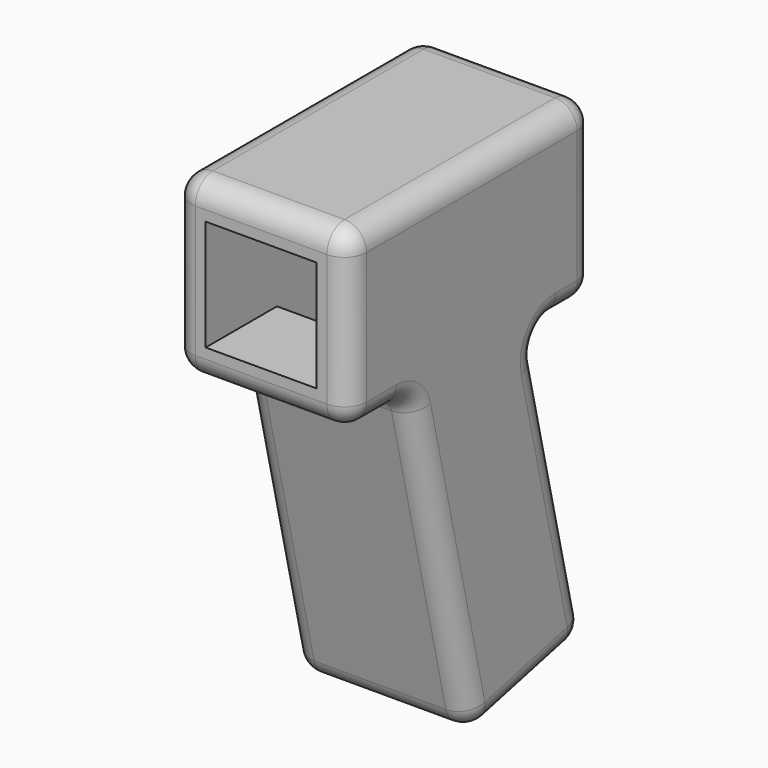
from build123d import *

# Parameters (mm, degrees)
F1_DEPTH      = 8
F2_W          = 10.1
F2_H          = 10.1
F3_DEPTH      = 28
F4_W          = 10.1
F4_H          = 10.1
F5_DEPTH      = 33.3776100313
F6_T1_DEPTH   = 16
F6_T3_DEPTH   = 12
F6_T5_DEPTH   = 24
F6_T7_DEPTH   = 19
F6_T9_DEPTH   = 23.6326677566
F6_T11_DEPTH  = 26
F6_S15_W      = 2
F6_S15_H      = 2
F6_T16_DEPTH  = 2
F6_S21_W      = 2
F6_S21_H      = 2
F6_T22_DEPTH  = 2
F6_S27_W      = 2
F6_S27_H      = 2
F6_T28_DEPTH  = 2
F6_S33_W      = 2
F6_S33_H      = 2
F6_T34_DEPTH  = 2
F6_T37_DEPTH  = 23.0526598256
F6_T39_DEPTH  = 2.4787085237
F6_T41_DEPTH  = 3.4135114731
F6_T43_DEPTH  = 27.1734272819
F6_S47_W      = 2
F6_S47_H      = 2
F6_T48_DEPTH  = 2
F6_S53_W      = 2
F6_S53_H      = 2
F6_T54_DEPTH  = 2
F6_S59_W      = 2
F6_S59_H      = 2
F6_T60_DEPTH  = 2
F6_T66_DEPTH  = 2
F6_T72_DEPTH  = 2
F6_S77_W      = 2
F6_S77_H      = 2
F6_T78_DEPTH  = 2
F6_S83_W      = 2
F6_S83_H      = 2
F6_T84_DEPTH  = 2
F6_S89_W      = 2
F6_S89_H      = 2
F6_T90_DEPTH  = 2
F6_T94_ANGLE  = 76.8460155346
F6_T96_ANGLE  = 103.1539844654
F6_T98_ANGLE  = 76.8460155346
F6_T100_ANGLE = 103.1539844654


# Not quite as in the source:
# - a fillet or chamfer that OpenCascade refuses, or shapes differently, is made with other operations: its cross-section is extruded or revolved along the edge and cut away or added


with BuildPart() as f1:
    # F0 (on Right) → F1 (new body, symmetric)
    with BuildSketch(Plane.YZ):
        Polygon((7, -8), (14, -8), (14, 8), (-14, 8), (-14, -8), (-7, -8), (0, -37.9528366029), (13.2749735829, -34.8504654882), align=None)
    extrude(amount=F1_DEPTH, both=True)

    # F2 (on face) → F3 (cut, through all)
    with BuildSketch(Plane(origin=(0, 14, 0), x_dir=(-1, 0, 0), z_dir=(0, 1, 0))):
        Rectangle(F2_W, F2_H)
    extrude(amount=-F3_DEPTH, mode=Mode.SUBTRACT)

    # F4 (on face) → F5 (cut, through all)
    with BuildSketch(Plane(origin=(0, 8.4102702856, -35.9873502358), x_dir=(1, 0, 0), z_dir=(0, 0.2275688933, -0.9737619826))):
        with Locations((0, 1.8205511468)):
            Rectangle(F4_W, F4_H)
    extrude(amount=-F5_DEPTH, mode=Mode.SUBTRACT)

    # F6: fillet of radius 2 on 24 edges, made by hand

    # F6_s2 → F6_t1 (join)
    with BuildSketch(Plane.YZ.offset(-8)):
        with BuildLine():
            ThreePointArc((-8.5864885269, -8), (-7.3435636646, -8.4331120695), (-6.6389645616, -9.5448622133))
            Line((-6.6389645616, -9.5448622133), (-7, -8))
            Line((-7, -8), (-8.5864885269, -8))
        make_face()
        with BuildLine():
            ThreePointArc((7.5737675111, -10.4551377867), (7.9544035458, -8.7570751377), (9.5212914763, -8))
            Line((9.5212914763, -8), (7, -8))
            Line((7, -8), (7.5737675111, -10.4551377867))
        make_face()
    extrude(amount=F6_T1_DEPTH)

    # F6_s4 → F6_t3 (cut)
    with BuildSketch(Plane.YZ.offset(-6)):
        with BuildLine():
            ThreePointArc((14, 6), (13.4142135624, 7.4142135624), (12, 8))
            Line((12, 8), (14, 8))
            Line((14, 8), (14, 6))
        make_face()
        with BuildLine():
            ThreePointArc((-12, 8), (-13.4142135624, 7.4142135624), (-14, 6))
            Line((-14, 6), (-14, 8))
            Line((-14, 8), (-12, 8))
        make_face()
    extrude(amount=F6_T3_DEPTH, mode=Mode.SUBTRACT)

    # F6_s6 → F6_t5 (cut)
    with BuildSketch(Plane.XZ.offset(-12)):
        with BuildLine():
            ThreePointArc((-8, 6), (-7.4142135624, 7.4142135624), (-6, 8))
            Line((-6, 8), (-8, 8))
            Line((-8, 8), (-8, 6))
        make_face()
        with BuildLine():
            ThreePointArc((8, 6), (7.4142135624, 7.4142135624), (6, 8))
            Line((6, 8), (8, 8))
            Line((8, 8), (8, 6))
        make_face()
    extrude(amount=F6_T5_DEPTH, mode=Mode.SUBTRACT)

    # F6_s8 → F6_t7 (cut)
    with BuildSketch(Plane.XY.offset(-13)):
        with BuildLine():
            ThreePointArc((-8, 12), (-7.4142135624, 13.4142135624), (-6, 14))
            Line((-6, 14), (-8, 14))
            Line((-8, 14), (-8, 12))
        make_face()
        with BuildLine():
            ThreePointArc((-8, -12), (-7.4142135624, -13.4142135624), (-6, -14))
            Line((-6, -14), (-8, -14))
            Line((-8, -14), (-8, -12))
        make_face()
        with BuildLine():
            ThreePointArc((8, 12), (7.4142135624, 13.4142135624), (6, 14))
            Line((6, 14), (8, 14))
            Line((8, 14), (8, 12))
        make_face()
        with BuildLine():
            ThreePointArc((8, -12), (7.4142135624, -13.4142135624), (6, -14))
            Line((6, -14), (8, -14))
            Line((8, -14), (8, -12))
        make_face()
    extrude(amount=F6_T7_DEPTH, mode=Mode.SUBTRACT)

    # F6_s10 → F6_t9 (cut)
    with BuildSketch(Plane(origin=(0, -13.2790801987, -3.1033308338), x_dir=(1, 0, 0), z_dir=(0, 0.9737619826, 0.2275688933))):
        with BuildLine():
            ThreePointArc((-6, 36.9570294162), (-7.4142135624, 36.3712429786), (-8, 34.9570294162))
            Line((-8, 34.9570294162), (-8, 36.9570294162))
            Line((-8, 36.9570294162), (-6, 36.9570294162))
        make_face()
        with BuildLine():
            ThreePointArc((6, 36.9570294162), (7.4142135624, 36.3712429786), (8, 34.9570294162))
            Line((8, 34.9570294162), (8, 36.9570294162))
            Line((8, 36.9570294162), (6, 36.9570294162))
        make_face()
    extrude(amount=F6_T9_DEPTH, mode=Mode.SUBTRACT)

    # F6_s12 → F6_t11 (cut)
    with BuildSketch(Plane.YZ.offset(-13)):
        with BuildLine():
            ThreePointArc((1.9475239652, -37.4976988162), (0.4371097915, -37.2491132687), (-0.4551377867, -36.0053126377))
            Line((-0.4551377867, -36.0053126377), (0, -37.9528366029))
            Line((0, -37.9528366029), (1.9475239652, -37.4976988162))
        make_face()
        with BuildLine():
            ThreePointArc((12.8198357962, -32.902941523), (12.5712502487, -34.4133556967), (11.3274496177, -35.3056032749))
            Line((11.3274496177, -35.3056032749), (13.2749735829, -34.8504654882))
            Line((13.2749735829, -34.8504654882), (12.8198357962, -32.902941523))
        make_face()
        with BuildLine():
            ThreePointArc((12, -8), (13.4142135624, -7.4142135624), (14, -6))
            Line((14, -6), (14, -8))
            Line((14, -8), (12, -8))
        make_face()
        with BuildLine():
            ThreePointArc((-14, -6), (-13.4142135624, -7.4142135624), (-12, -8))
            Line((-12, -8), (-14, -8))
            Line((-14, -8), (-14, -6))
        make_face()
    extrude(amount=F6_T11_DEPTH, mode=Mode.SUBTRACT)


with BuildPart() as f6_tool14:
    # F6_s15 → F6_t16 (new body)
    with BuildSketch(Plane.XZ.offset(-12)):
        with Locations((-7, 7)):
            Rectangle(F6_S15_W, F6_S15_H)
    extrude(amount=-F6_T16_DEPTH)

    # F6_s17 → F6_t18 (revolve, cut)
    with BuildSketch(Plane(origin=(-6, 12, 6), x_dir=(0.7071067812, 0, -0.7071067812), z_dir=(0.7071067812, 0, 0.7071067812))):
        with BuildLine():
            ThreePointArc((0, -2), (2, 0), (0, 2))
            Line((0, 2), (0, -2))
        make_face()
    revolve(axis=Axis((-6, 12, 6), (0, 1, 0)), mode=Mode.SUBTRACT)


with BuildPart() as f1_1:
    add(f1.part)

    # F6_t13: cut F6_tool14
    add(f6_tool14.part, mode=Mode.SUBTRACT)


with BuildPart() as f6_tool20:
    # F6_s21 → F6_t22 (new body)
    with BuildSketch(Plane.YZ.offset(6)):
        with Locations((13, 7)):
            Rectangle(F6_S21_W, F6_S21_H)
    extrude(amount=F6_T22_DEPTH)

    # F6_s23 → F6_t24 (revolve, cut)
    with BuildSketch(Plane(origin=(6, 12, 6), x_dir=(0, -0.7071067812, -0.7071067812), z_dir=(0, -0.7071067812, 0.7071067812))):
        with BuildLine():
            ThreePointArc((0, -2), (2, 0), (0, 2))
            Line((0, 2), (0, -2))
        make_face()
    revolve(axis=Axis((6, 12, 6), (1, 0, 0)), mode=Mode.SUBTRACT)


with BuildPart() as f1_2:
    add(f1_1.part)

    # F6_t19: cut F6_tool20
    add(f6_tool20.part, mode=Mode.SUBTRACT)


with BuildPart() as f6_tool26:
    # F6_s27 → F6_t28 (new body)
    with BuildSketch(Plane.XZ.offset(12)):
        with Locations((-7, 7)):
            Rectangle(F6_S27_W, F6_S27_H)
    extrude(amount=F6_T28_DEPTH)

    # F6_s29 → F6_t30 (revolve, cut)
    with BuildSketch(Plane(origin=(-6, -12, 6), x_dir=(0.7071067812, 0, -0.7071067812), z_dir=(-0.7071067812, 0, -0.7071067812))):
        with BuildLine():
            ThreePointArc((0, -2), (2, 0), (0, 2))
            Line((0, 2), (0, -2))
        make_face()
    revolve(axis=Axis((-6, -12, 6), (0, -1, 0)), mode=Mode.SUBTRACT)


with BuildPart() as f1_3:
    add(f1_2.part)

    # F6_t25: cut F6_tool26
    add(f6_tool26.part, mode=Mode.SUBTRACT)


with BuildPart() as f6_tool32:
    # F6_s33 → F6_t34 (new body)
    with BuildSketch(Plane.YZ.offset(6)):
        with Locations((-13, 7)):
            Rectangle(F6_S33_W, F6_S33_H)
    extrude(amount=F6_T34_DEPTH)

    # F6_s35 → F6_t36 (revolve, cut)
    with BuildSketch(Plane(origin=(6, -12, 6), x_dir=(0, 0.7071067812, -0.7071067812), z_dir=(0, -0.7071067812, -0.7071067812))):
        with BuildLine():
            ThreePointArc((0, -2), (2, 0), (0, 2))
            Line((0, 2), (0, -2))
        make_face()
    revolve(axis=Axis((6, -12, 6), (1, 0, 0)), mode=Mode.SUBTRACT)


with BuildPart() as f1_4:
    add(f1_3.part)

    # F6_t31: cut F6_tool32
    add(f6_tool32.part, mode=Mode.SUBTRACT)

    # F6_s38 → F6_t37 (cut)
    with BuildSketch(Plane(origin=(0, 7.9551324989, -34.0398262706), x_dir=(1, 0, 0), z_dir=(0, -0.2275688933, 0.9737619826))):
        with BuildLine():
            ThreePointArc((-6, 4.9957827315), (-7.4142135624, 4.4099962939), (-8, 2.9957827315))
            Line((-8, 2.9957827315), (-8, 4.9957827315))
            Line((-8, 4.9957827315), (-6, 4.9957827315))
        make_face()
        with BuildLine():
            ThreePointArc((6, 4.9957827315), (7.4142135624, 4.4099962939), (8, 2.9957827315))
            Line((8, 2.9957827315), (8, 4.9957827315))
            Line((8, 4.9957827315), (6, 4.9957827315))
        make_face()
    extrude(amount=F6_T37_DEPTH, mode=Mode.SUBTRACT)

    # F6_s40 → F6_t39 (cut)
    with BuildSketch(Plane.XZ.offset(-12)):
        with BuildLine():
            ThreePointArc((-8, -6), (-7.4142135624, -7.4142135624), (-6, -8))
            Line((-6, -8), (-8, -8))
            Line((-8, -8), (-8, -6))
        make_face()
        with BuildLine():
            ThreePointArc((8, -6), (7.4142135624, -7.4142135624), (6, -8))
            Line((6, -8), (8, -8))
            Line((8, -8), (8, -6))
        make_face()
    extrude(amount=F6_T39_DEPTH, mode=Mode.SUBTRACT)

    # F6_s42 → F6_t41 (cut)
    with BuildSketch(Plane.XZ.offset(8.5864885269)):
        with BuildLine():
            ThreePointArc((-8, -6), (-7.4142135624, -7.4142135624), (-6, -8))
            Line((-6, -8), (-8, -8))
            Line((-8, -8), (-8, -6))
        make_face()
        with BuildLine():
            ThreePointArc((8, -6), (7.4142135624, -7.4142135624), (6, -8))
            Line((6, -8), (8, -8))
            Line((8, -8), (8, -6))
        make_face()
    extrude(amount=F6_T41_DEPTH, mode=Mode.SUBTRACT)

    # F6_s44 → F6_t43 (cut)
    with BuildSketch(Plane(origin=(0, 1.771305724, -7.5793758462), x_dir=(1, 0, 0), z_dir=(0, 0.2275688933, -0.9737619826))):
        with BuildLine():
            ThreePointArc((-8, 6.6368850251), (-7.4142135624, 8.0510985874), (-6, 8.6368850251))
            Line((-6, 8.6368850251), (-8, 8.6368850251))
            Line((-8, 8.6368850251), (-8, 6.6368850251))
        make_face()
        with BuildLine():
            ThreePointArc((8, 6.6368850251), (7.4142135624, 8.0510985874), (6, 8.6368850251))
            Line((6, 8.6368850251), (8, 8.6368850251))
            Line((8, 8.6368850251), (8, 6.6368850251))
        make_face()
    extrude(amount=F6_T43_DEPTH, mode=Mode.SUBTRACT)


with BuildPart() as f6_tool46:
    # F6_s47 → F6_t48 (new body)
    with BuildSketch(Plane.YZ.offset(6)):
        with Locations((-13, -7)):
            Rectangle(F6_S47_W, F6_S47_H)
    extrude(amount=F6_T48_DEPTH)

    # F6_s49 → F6_t50 (revolve, cut)
    with BuildSketch(Plane(origin=(6, -12, -6), x_dir=(0, 0.7071067812, 0.7071067812), z_dir=(0, 0.7071067812, -0.7071067812))):
        with BuildLine():
            ThreePointArc((0, -2), (2, 0), (0, 2))
            Line((0, 2), (0, -2))
        make_face()
    revolve(axis=Axis((6, -12, -6), (1, 0, 0)), mode=Mode.SUBTRACT)


with BuildPart() as f1_5:
    add(f1_4.part)

    # F6_t45: cut F6_tool46
    add(f6_tool46.part, mode=Mode.SUBTRACT)


with BuildPart() as f6_tool52:
    # F6_s53 → F6_t54 (new body)
    with BuildSketch(Plane.YZ.offset(6)):
        with Locations((13, -7)):
            Rectangle(F6_S53_W, F6_S53_H)
    extrude(amount=F6_T54_DEPTH)

    # F6_s55 → F6_t56 (revolve, cut)
    with BuildSketch(Plane(origin=(6, 12, -6), x_dir=(0, -0.7071067812, 0.7071067812), z_dir=(0, 0.7071067812, 0.7071067812))):
        with BuildLine():
            ThreePointArc((0, -2), (2, 0), (0, 2))
            Line((0, 2), (0, -2))
        make_face()
    revolve(axis=Axis((6, 12, -6), (1, 0, 0)), mode=Mode.SUBTRACT)


with BuildPart() as f1_6:
    add(f1_5.part)

    # F6_t51: cut F6_tool52
    add(f6_tool52.part, mode=Mode.SUBTRACT)


with BuildPart() as f6_tool58:
    # F6_s59 → F6_t60 (new body)
    with BuildSketch(Plane(origin=(0, 2.9171793321, 0.6817469609), x_dir=(1, 0, 0), z_dir=(0, 0.9737619826, 0.2275688933))):
        with Locations((7, 35.9570294162)):
            Rectangle(F6_S59_W, F6_S59_H)
    extrude(amount=F6_T60_DEPTH)

    # F6_s61 → F6_t62 (revolve, cut)
    with BuildSketch(Plane(origin=(6, 10.872311831, -33.3580793097), x_dir=(-0.7071067812, -0.1609155077, 0.6885537012), z_dir=(-0.7071067812, 0.1609155077, -0.6885537012))):
        with BuildLine():
            ThreePointArc((0, -2), (2, 0), (0, 2))
            Line((0, 2), (0, -2))
        make_face()
    revolve(axis=Axis((6, 10.872311831, -33.3580793097), (0, 0.9737619826, 0.2275688933)), mode=Mode.SUBTRACT)


with BuildPart() as f1_7:
    add(f1_6.part)

    # F6_t57: cut F6_tool58
    add(f6_tool58.part, mode=Mode.SUBTRACT)


with BuildPart() as f6_tool64:
    # F6_s65 → F6_t66 (new body)
    with BuildSketch(Plane.YZ.offset(6)):
        Polygon((1.4923861785, -35.550174851), (-0.4551377867, -36.0053126377), (0, -37.9528366029), (1.9475239652, -37.4976988162), align=None)
    extrude(amount=F6_T66_DEPTH)

    # F6_s67 → F6_t68 (revolve, cut)
    with BuildSketch(Plane(origin=(6, 1.4923861785, -35.550174851), x_dir=(0, 0.5276381935, 0.8494692088), z_dir=(0, 0.8494692088, -0.5276381935))):
        with BuildLine():
            ThreePointArc((0, -2), (2, 0), (0, 2))
            Line((0, 2), (0, -2))
        make_face()
    revolve(axis=Axis((6, 1.4923861785, -35.550174851), (1, 0, 0)), mode=Mode.SUBTRACT)


with BuildPart() as f1_8:
    add(f1_7.part)

    # F6_t63: cut F6_tool64
    add(f6_tool64.part, mode=Mode.SUBTRACT)


with BuildPart() as f6_tool70:
    # F6_s71 → F6_t72 (new body)
    with BuildSketch(Plane.YZ.offset(-6)):
        Polygon((1.4923861785, -35.550174851), (-0.4551377867, -36.0053126377), (0, -37.9528366029), (1.9475239652, -37.4976988162), align=None)
    extrude(amount=-F6_T72_DEPTH)

    # F6_s73 → F6_t74 (revolve, cut)
    with BuildSketch(Plane(origin=(-6, 1.4923861785, -35.550174851), x_dir=(0, 0.5276381935, 0.8494692088), z_dir=(0, -0.8494692088, 0.5276381935))):
        with BuildLine():
            ThreePointArc((0, -2), (2, 0), (0, 2))
            Line((0, 2), (0, -2))
        make_face()
    revolve(axis=Axis((-6, 1.4923861785, -35.550174851), (-1, 0, 0)), mode=Mode.SUBTRACT)


with BuildPart() as f1_9:
    add(f1_8.part)

    # F6_t69: cut F6_tool70
    add(f6_tool70.part, mode=Mode.SUBTRACT)


with BuildPart() as f6_tool76:
    # F6_s77 → F6_t78 (new body)
    with BuildSketch(Plane.YZ.offset(-6)):
        with Locations((-13, -7)):
            Rectangle(F6_S77_W, F6_S77_H)
    extrude(amount=-F6_T78_DEPTH)

    # F6_s79 → F6_t80 (revolve, cut)
    with BuildSketch(Plane(origin=(-6, -12, -6), x_dir=(0, 0.7071067812, 0.7071067812), z_dir=(0, -0.7071067812, 0.7071067812))):
        with BuildLine():
            ThreePointArc((0, -2), (2, 0), (0, 2))
            Line((0, 2), (0, -2))
        make_face()
    revolve(axis=Axis((-6, -12, -6), (-1, 0, 0)), mode=Mode.SUBTRACT)


with BuildPart() as f1_10:
    add(f1_9.part)

    # F6_t75: cut F6_tool76
    add(f6_tool76.part, mode=Mode.SUBTRACT)


with BuildPart() as f6_tool82:
    # F6_s83 → F6_t84 (new body)
    with BuildSketch(Plane.YZ.offset(-6)):
        with Locations((13, -7)):
            Rectangle(F6_S83_W, F6_S83_H)
    extrude(amount=-F6_T84_DEPTH)

    # F6_s85 → F6_t86 (revolve, cut)
    with BuildSketch(Plane(origin=(-6, 12, -6), x_dir=(0, -0.7071067812, 0.7071067812), z_dir=(0, -0.7071067812, -0.7071067812))):
        with BuildLine():
            ThreePointArc((0, -2), (2, 0), (0, 2))
            Line((0, 2), (0, -2))
        make_face()
    revolve(axis=Axis((-6, 12, -6), (-1, 0, 0)), mode=Mode.SUBTRACT)


with BuildPart() as f1_11:
    add(f1_10.part)

    # F6_t81: cut F6_tool82
    add(f6_tool82.part, mode=Mode.SUBTRACT)


with BuildPart() as f6_tool88:
    # F6_s89 → F6_t90 (new body)
    with BuildSketch(Plane(origin=(0, 2.9171793321, 0.6817469609), x_dir=(1, 0, 0), z_dir=(0, 0.9737619826, 0.2275688933))):
        with Locations((-7, 35.9570294162)):
            Rectangle(F6_S89_W, F6_S89_H)
    extrude(amount=F6_T90_DEPTH)

    # F6_s91 → F6_t92 (revolve, cut)
    with BuildSketch(Plane(origin=(-6, 10.872311831, -33.3580793097), x_dir=(0.7071067812, -0.1609155077, 0.6885537012), z_dir=(-0.7071067812, -0.1609155077, 0.6885537012))):
        with BuildLine():
            ThreePointArc((0, -2), (2, 0), (0, 2))
            Line((0, 2), (0, -2))
        make_face()
    revolve(axis=Axis((-6, 10.872311831, -33.3580793097), (0, 0.9737619826, 0.2275688933)), mode=Mode.SUBTRACT)


with BuildPart() as f1_12:
    add(f1_11.part)

    # F6_t87: cut F6_tool88
    add(f6_tool88.part, mode=Mode.SUBTRACT)

    # F6_s93 → F6_t94 (revolve, cut)
    with BuildSketch(Plane.XZ.offset(8.5864885269)):
        with BuildLine():
            ThreePointArc((8, -6), (7.4142135624, -7.4142135624), (6, -8))
            Line((6, -8), (8, -8))
            Line((8, -8), (8, -6))
        make_face()
    revolve(axis=Axis((8, -8.5864885269, -10), (-1, 0, 0)), revolution_arc=F6_T94_ANGLE, mode=Mode.SUBTRACT)

    # F6_s95 → F6_t96 (revolve, cut)
    with BuildSketch(Plane(origin=(0, 2.7090642137, -11.5920225343), x_dir=(1, 0, 0), z_dir=(0, 0.2275688933, -0.9737619826))):
        with BuildLine():
            ThreePointArc((8, -2.9957827315), (7.4142135624, -4.4099962939), (6, -4.9957827315))
            Line((6, -4.9957827315), (8, -4.9957827315))
            Line((8, -4.9957827315), (8, -2.9957827315))
        make_face()
    revolve(axis=Axis((8, 9.5212914763, -10), (-1, 0, 0)), revolution_arc=F6_T96_ANGLE, mode=Mode.SUBTRACT)

    # F6_s97 → F6_t98 (revolve, cut)
    with BuildSketch(Plane.XZ.offset(8.5864885269)):
        with BuildLine():
            ThreePointArc((-8, -6), (-7.4142135624, -7.4142135624), (-6, -8))
            Line((-6, -8), (-8, -8))
            Line((-8, -8), (-8, -6))
        make_face()
    revolve(axis=Axis((-8, -8.5864885269, -10), (-1, 0, 0)), revolution_arc=F6_T98_ANGLE, mode=Mode.SUBTRACT)

    # F6_s99 → F6_t100 (revolve, cut)
    with BuildSketch(Plane(origin=(0, 2.7090642137, -11.5920225343), x_dir=(1, 0, 0), z_dir=(0, 0.2275688933, -0.9737619826))):
        with BuildLine():
            ThreePointArc((-6, -4.9957827315), (-7.4142135624, -4.4099962939), (-8, -2.9957827315))
            Line((-8, -2.9957827315), (-8, -4.9957827315))
            Line((-8, -4.9957827315), (-6, -4.9957827315))
        make_face()
    revolve(axis=Axis((-8, 9.5212914763, -10), (-1, 0, 0)), revolution_arc=F6_T100_ANGLE, mode=Mode.SUBTRACT)


solid = f1_12.part
